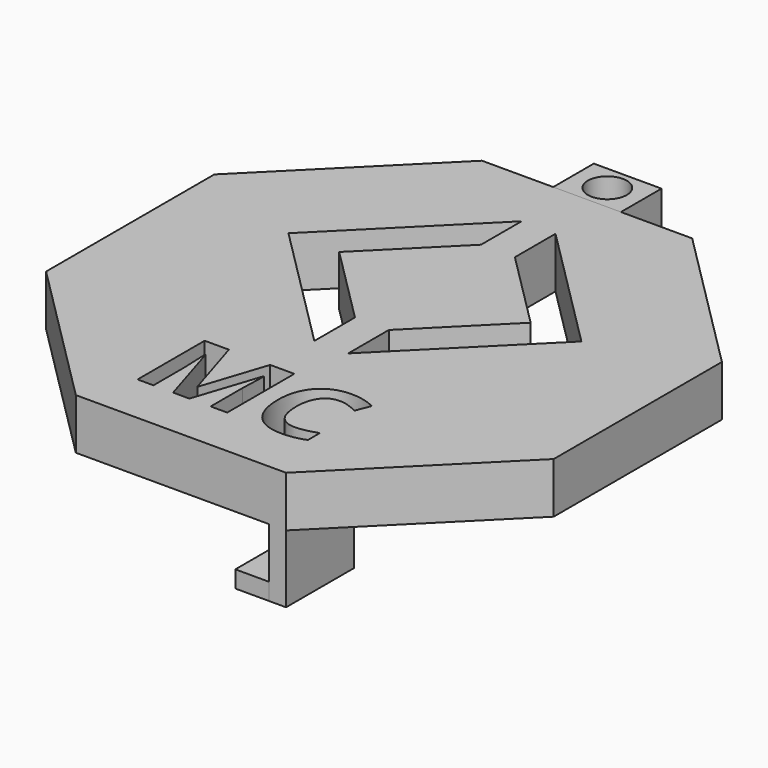
from build123d import *

# Parameters (mm, degrees)
F1_DEPTH     = 3
F2_TEXT_SIZE = 6.9444444444
F3_DEPTH     = 3.001
F4_W         = 1
F4_H         = 5
F5_DEPTH     = 4
F6_W         = 5
F6_H         = 1
F7_DEPTH     = 2
F8_W         = 4
F8_H         = 3
F9_DEPTH     = 3
F10_R        = 1.15
F11_DEPTH    = 3.0010001


# Not quite as in the source:
# - Text() gives the source's letters only with a copy of the font that has no kerning and outlines rounded to 1/6400 em; it was checked with that copy


with BuildPart() as f1:
    # F0 (on Top) → F1 (new body)
    with BuildSketch(Plane.XY):
        Polygon((15, -6.2132034356), (15, 6.2132034356), (6.2132034356, 15), (-6.2132034356, 15), (-15, 6.2132034356), (-15, -6.2132034356), (-6.2132034356, -15), (6.2132034356, -15), align=None)
    extrude(amount=F1_DEPTH)

    # F2 (on face) → F3 (cut, through all)
    with BuildSketch(Plane.XY.offset(3)):
        Polygon((1, 8.418436326), (5.6568542495, 3.7615820765), (1, -0.8952721729), (1, -3.8952721729), (8.6568542495, 3.7615820765), (1, 11.418436326), align=None)
        Polygon((-1, -0.8952721729), (-5.6568542495, 3.7615820765), (-1, 8.418436326), (-1, 11.418436326), (-8.6568542495, 3.7615820765), (-1, -3.8952721729), align=None)
        with Locations((-5.5891927083, -12)):
            Text('MC', F2_TEXT_SIZE, font='Open Sans', font_style=FontStyle.BOLD, text_align=(TextAlign.LEFT, TextAlign.BOTTOM))
    extrude(amount=-F3_DEPTH, mode=Mode.SUBTRACT)

    # F4 (on face) → F5 (join)
    with BuildSketch(Plane(origin=(0, 0, 0), x_dir=(1, 0, 0), z_dir=(0, 0, -1))):
        with Locations((5.7132034356, 12.5)):
            Rectangle(F4_W, F4_H)
    extrude(amount=F5_DEPTH)


with BuildPart() as f7:
    # F6 (on face) → F7 (new body)
    with BuildSketch(Plane(origin=(5.2132034356, 0, 0), x_dir=(0, -1, 0), z_dir=(-1, 0, 0))):
        with Locations((12.5, -3.5)):
            Rectangle(F6_W, F6_H)
    extrude(amount=F7_DEPTH)


with BuildPart() as f9:
    # F8 (on face) → F9 (new body)
    with BuildSketch(Plane(origin=(0, 15, 0), x_dir=(-1, 0, 0), z_dir=(0, 1, 0))):
        with Locations((0, 1.5)):
            Rectangle(F8_W, F8_H)
    extrude(amount=F9_DEPTH)

    # F10 (on face) → F11 (cut, through all)
    with BuildSketch(Plane(origin=(0, 0, 0), x_dir=(1, 0, 0), z_dir=(0, 0, -1))):
        with Locations((0, -16.5)):
            Circle(F10_R)
    extrude(amount=-F11_DEPTH, mode=Mode.SUBTRACT)


solid = Compound([f1.part, f7.part, f9.part])
